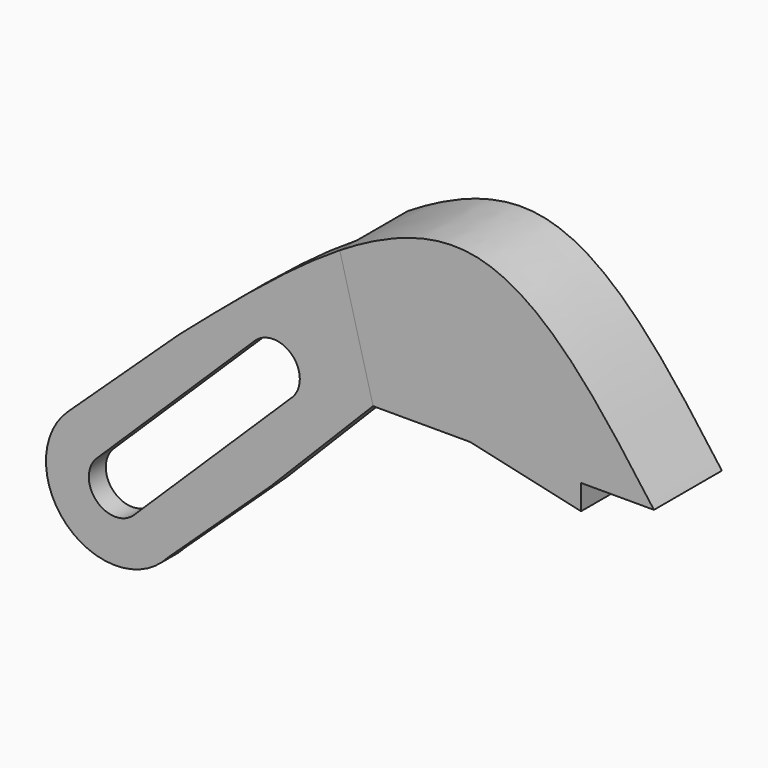
from build123d import *

# Parameters (mm, degrees)
F1_DEPTH = 8
F2_DEPTH = 2
F3_DEPTH = 25


with BuildPart() as f1:
    # F0 (on Front) → F1 (new body)
    with BuildSketch(Plane.XZ):
        with BuildLine():
            Line((-6.8668625318, 0), (0, 0))
            add(Edge.make_bspline(
                [(0, 0), (-5.5166817517, 7.5273476461), (-13.9427053961, 19.0244054975), (-25.4283193392, 14.4964589712), (-29.5906448635, 11.9035035184)],
                knots=[0, 0, 0, 0, 0.4664815309, 0.7124906939, 0.7124906939, 0.7124906939, 0.7124906939], degree=3))
            Line((-29.5906448635, 11.9035035184), (-26.4566000551, 0))
            Line((-26.4566000551, 0), (-17.324373126, 0))
            Line((-17.324373126, 0), (-6.8668625318, -2.3509128803))
            Line((-6.8668625318, -2.3509128803), (-6.8668625318, 0))
        make_face()
        Polygon((0, -3.8946259301), (0, 0), (-6.8668625318, 0), (-6.8668625318, -2.3509128803), align=None)
    extrude(amount=-F1_DEPTH)

    # F0 (on Front) → F3 (cut)
    with BuildSketch(Plane.XZ):
        Polygon((0, -3.8946259301), (0, 0), (-6.8668625318, 0), (-6.8668625318, -2.3509128803), align=None)
    extrude(amount=-F3_DEPTH, mode=Mode.SUBTRACT)


with BuildPart() as f2:
    # F0 (on Front) → F2 (new body)
    with BuildSketch(Plane.XZ):
        with BuildLine():
            Line((-26.4566000551, 0), (-29.5906448635, 11.9035035184))
            add(Edge.make_bspline(
                [(-29.5906448635, 11.9035035184), (-34.4551275869, 8.8731333733), (-39.5880898188, 4.4365666867), (-44.7210520506, 0)],
                knots=[0.7124906939, 0.7124906939, 0.7124906939, 0.7124906939, 1, 1, 1, 1], degree=3))
            Line((-44.7210520506, 0), (-55.1962554455, -9.8037142307))
            ThreePointArc((-55.1962554455, -9.8037142307), (-55.2651318504, -19.2779776557), (-45.7999520147, -18.85752304))
            Line((-45.7999520147, -18.85752304), (-36.1260175705, -9.8037142307))
            Line((-36.1260175705, -9.8037142307), (-26.4566000551, 0))
        make_face()
        with BuildLine():
            ThreePointArc((-34.0009998268, -1.6744260512), (-34.1076420427, -1.7855743191), (-34.2209268371, -1.8899441183))
            Line((-34.2209268371, -1.8899441183), (-48.9028869032, -16.2775705017))
            ThreePointArc((-48.9028869032, -16.2775705017), (-48.9824013436, -16.359123751), (-49.065547898, -16.4369705825))
            ThreePointArc((-49.065547898, -16.4369705825), (-52.6027386022, -16.2321661604), (-52.3827507862, -12.6958872842))
            Line((-52.3827507862, -12.6958872842), (-37.6682687749, 1.7236090672))
            ThreePointArc((-37.6682687749, 1.7236090672), (-37.6071987867, 1.7855743191), (-37.5440096809, 1.8453771016))
            ThreePointArc((-37.5440096809, 1.8453771016), (-34.095471429, 1.7735658352), (-34.0009998268, -1.6744260512))
        make_face(mode=Mode.SUBTRACT)
    extrude(amount=-F2_DEPTH)


solid = Compound([f1.part, f2.part])
